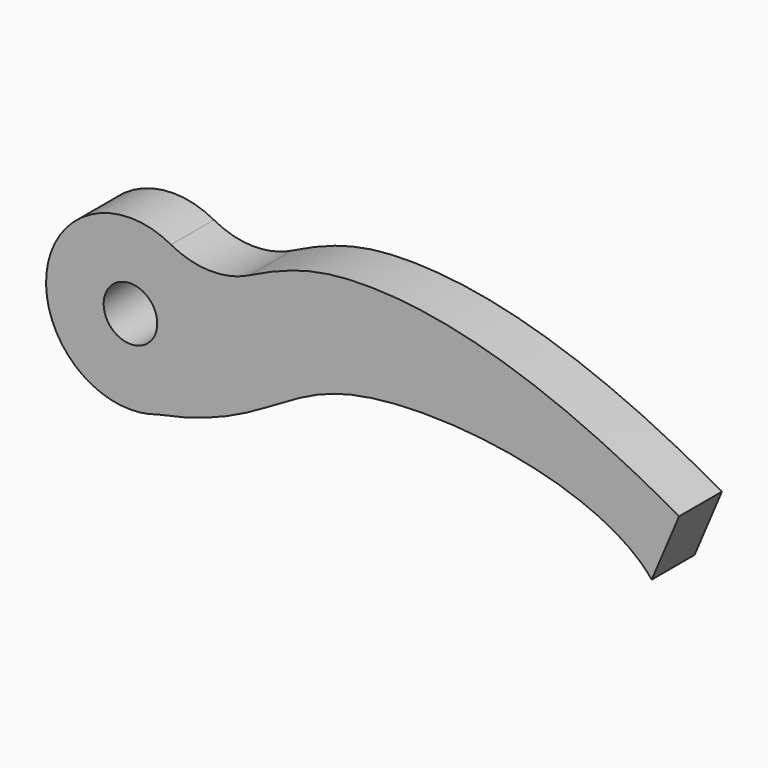
from build123d import *

# Parameters (mm, degrees)
F1_DEPTH = 3.175
F2_R     = 5


# Not quite as in the source:
# - a length typed as a fraction of an inch, garbled in the dataset ("3 / 203.2 mm" for 3/8 in), is restored


with BuildPart() as f1:
    # F0 (on Front) → F1 (new body)
    with BuildSketch(Plane.XZ):
        with BuildLine():
            ThreePointArc((5, 0), (4.7976890268, 1.4078991449), (4.2071279991, 2.7018649113))
            ThreePointArc((4.2071279991, 2.7018649113), (0.0116152193, 4.9999865086), (-4.1945295238, 2.7213823829))
            ThreePointArc((-4.1945295238, 2.7213823829), (-4.3935698421, -2.3867433969), (0, -5))
            add(Edge.make_bspline(
                [(0, -5), (0.5720738613, -4.9218364583), (1.1062852924, -4.8328629446), (1.6070336906, -4.7347061912)],
                knots=[0, 0, 0, 0, 0.0353074902, 0.0353074902, 0.0353074902, 0.0353074902], degree=3))
            ThreePointArc((1.6070336906, -4.7347061912), (3.070488906, -3.9461497536), (4.1945295238, -2.7213823829))
            ThreePointArc((4.1945295238, -2.7213823829), (4.7944054699, -1.4190405881), (5, 0))
        make_face()
        with BuildLine():
            ThreePointArc((1.3244951977, 0.8751392582), (1.5203276582, 0.4569026831), (1.5875, 0))
            ThreePointArc((1.5875, 0), (-1.5203276582, -0.4569026831), (1.3244951977, 0.8751392582))
        make_face(mode=Mode.SUBTRACT)
        with BuildLine():
            add(Edge.make_bspline(
                [(4.2071279991, 2.7018649113), (8.5330066632, 5.3268453963), (13.9608292527, 6.9611647512), (24.1781340673, 4.7387528577), (32.5091555715, 0)],
                knots=[0.1019845344, 0.1019845344, 0.1019845344, 0.1019845344, 0.46554979, 1, 1, 1, 1], degree=3))
            ThreePointArc((4.2071279991, 2.7018649113), (4.7976890268, 1.4078991449), (5, 0))
            ThreePointArc((5, 0), (4.7944054699, -1.4190405881), (4.1945295238, -2.7213823829))
            ThreePointArc((4.1945295238, -2.7213823829), (3.070488906, -3.9461497536), (1.6070336906, -4.7347061912))
            add(Edge.make_bspline(
                [(1.6070336906, -4.7347061912), (7.7069500406, -3.5389999501), (10.2510979188, 2.1993831398), (27.8217853485, 0), (30.8888312429, -3.8289688528)],
                knots=[0.0353074902, 0.0353074902, 0.0353074902, 0.0353074902, 0.4654091895, 1, 1, 1, 1], degree=3))
            Line((30.8888312429, -3.8289688528), (32.5091555715, 0))
        make_face()
        with BuildLine():
            add(Edge.make_bspline(
                [(0, -5), (0.5720738613, -4.9218364583), (1.1062852924, -4.8328629446), (1.6070336906, -4.7347061912)],
                knots=[0, 0, 0, 0, 0.0353074902, 0.0353074902, 0.0353074902, 0.0353074902], degree=3))
            ThreePointArc((0, -5), (0.814392118, -4.9332307343), (1.6070336906, -4.7347061912))
        make_face()
    extrude(amount=F1_DEPTH)

    # F2
    f2_edges = [f1.edges().sort_by_distance(p)[0] for p in [
        (4.207128, -1.5875, 2.701865),
    ]]
    fillet(f2_edges, radius=F2_R)


solid = f1.part
